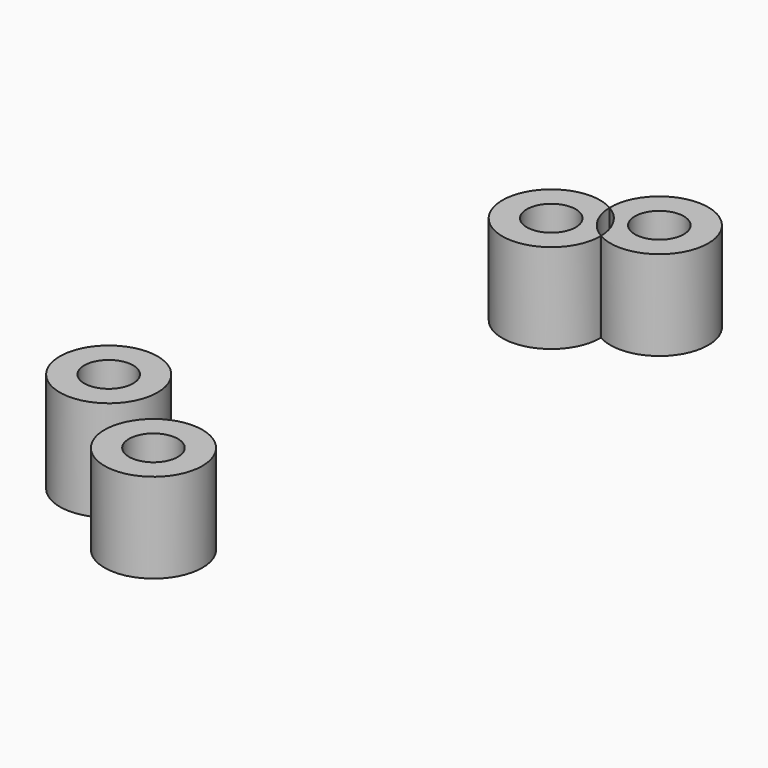
from build123d import *

# Parameters (mm, degrees)
F0_R     = 6
F1_DEPTH = 22
F0_R_2   = 12
F2_DEPTH = 24.7


# Not quite as in the source:
# - a feature names something its author has since deleted; it is built from what else it names


with BuildPart() as f1:
    # F0 (on Top) → F1 (new body)
    with BuildSketch(Plane.XY):
        with BuildLine():
            ThreePointArc((-22.3394160141, 61.2613618045), (-26.6720359479, 65.5415552979), (-28.3454602985, 71.3974329242))
            ThreePointArc((-28.3454602985, 71.3974329242), (-44.7263073816, 54.9955562097), (-22.3365694268, 61))
            ThreePointArc((-22.3365694268, 61), (-22.3372810947, 61.1306886528), (-22.3394160141, 61.2613618045))
        make_face()
        with Locations((-34.3365694268, 61)):
            Circle(F0_R, mode=Mode.SUBTRACT)
    extrude(amount=F1_DEPTH)


with BuildPart() as f1b:
    # F0 (on Top) → F1, piece 2 (new body)
    with BuildSketch(Plane.XY):
        with Locations((-34.3365694268, -61)):
            Circle(F0_R_2)
        with Locations((-34.3365694268, -61)):
            Circle(F0_R, mode=Mode.SUBTRACT)
    extrude(amount=F1_DEPTH)


with BuildPart() as f1c:
    # F0 (on Top) → F1, piece 3 (new body)
    with BuildSketch(Plane.XY):
        with BuildLine():
            ThreePointArc((-22.3394160141, 61.2613618045), (-10.3438630956, 61.2690567739), (-4.3483068859, 71.6587947287))
            ThreePointArc((-4.3483068859, 71.6587947287), (-16.4789955387, 83.6580830607), (-28.3454602985, 71.3974329242))
            ThreePointArc((-28.3454602985, 71.3974329242), (-24.0128403647, 67.1172394308), (-22.3394160141, 61.2613618045))
        make_face()
        with Locations((-16.3483068859, 71.6587947287)):
            Circle(F0_R, mode=Mode.SUBTRACT)
    extrude(amount=F1_DEPTH)


with BuildPart() as f2:
    # F0 (on Top) → F2 (new body)
    with BuildSketch(Plane.XY):
        with Locations((-56.8374801716, -46.6020476776)):
            Circle(F0_R_2)
        with Locations((-56.8374801716, -46.6020476776)):
            Circle(F0_R, mode=Mode.SUBTRACT)
    extrude(amount=F2_DEPTH)


solid = Compound([f1.part, f1b.part, f1c.part, f2.part])
